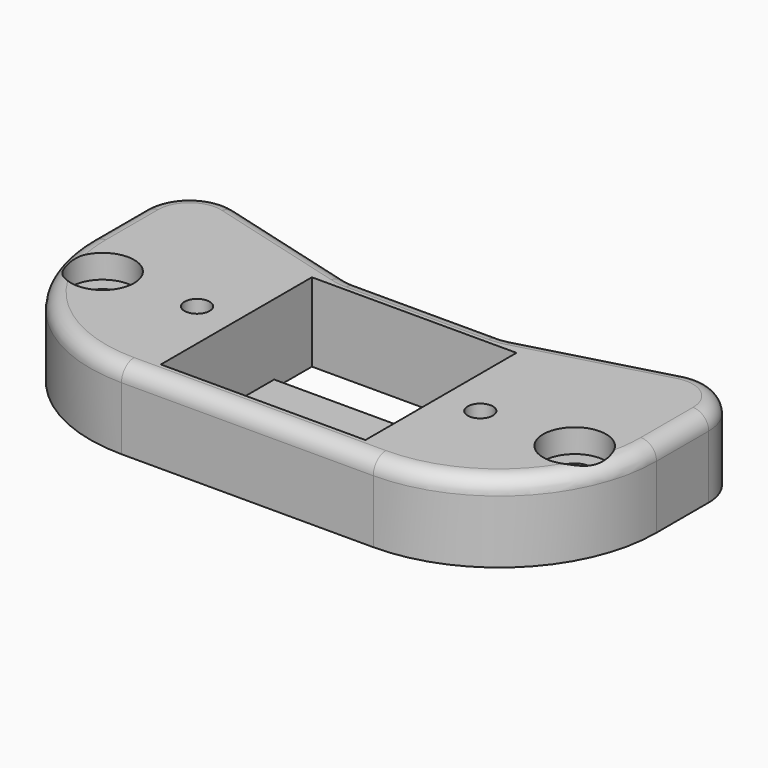
from build123d import *

# Parameters (mm, degrees)
F0_R           = 0.8
F0_W           = 13
F0_H           = 12
F1_DEPTH       = 5
F2_W           = 13
F2_H           = 6
F3_DEPTH       = 0.5
F5_D           = 2
F5_DEPTH       = 20
F5_CBORE_D     = 4
F5_CBORE_DEPTH = 1.5
F5_TIP         = 0.600860619
F6_R           = 10
F7_R           = 3
F8_T1_DEPTH    = 4.1430571099
F8_T3_DEPTH    = 9.217139142
F8_T5_DEPTH    = 16
F8_T7_DEPTH    = 9.0537269763
F8_T9_DEPTH    = 9.217139142
F8_T12_ANGLE   = 90
F8_T14_ANGLE   = 105.2904097565
F8_T16_ANGLE   = 90
F8_T18_ANGLE   = 15.2904100724
F8_T20_ANGLE   = 15.2904100724
F8_T22_ANGLE   = 105.2904094573


# Not quite as in the source:
# - a fillet or chamfer that OpenCascade refuses, or shapes differently, is made with other operations: its cross-section is extruded or revolved along the edge and cut away or added


with BuildPart() as f1:
    # F0 (on Top) → F1 (new body)
    with BuildSketch(Plane.XY):
        Polygon((-18, -7.25), (18, -7.25), (18, 7.25), (4.9295582736, 7.25), (-4.9295582736, 7.25), (-18, 7.25), align=None)
        with Locations((-9, 0)):
            Circle(F0_R, mode=Mode.SUBTRACT)
        Rectangle(F0_W, F0_H, mode=Mode.SUBTRACT)
        with Locations((9, 0)):
            Circle(F0_R, mode=Mode.SUBTRACT)
        with BuildLine():
            Line((4.9295582736, 7.25), (18, 7.25))
            ThreePointArc((18, 7.25), (17.6073787038, 9), (16.5047771245, 10.4145392323))
            Line((16.5047771245, 10.4145392323), (4.9295582736, 7.25))
        make_face()
        with BuildLine():
            ThreePointArc((-16.5047771245, 10.4145392323), (-17.6073787038, 9), (-18, 7.25))
            Line((-18, 7.25), (-4.9295582736, 7.25))
            Line((-4.9295582736, 7.25), (-16.5047771245, 10.4145392323))
        make_face()
    extrude(amount=F1_DEPTH)

    # F2 (on face) → F3 (join)
    with BuildSketch(Plane(origin=(0, 0, 0), x_dir=(1, 0, 0), z_dir=(0, 0, -1))):
        Rectangle(F2_W, F2_H)
    extrude(amount=-F3_DEPTH)

    # F5
    with Locations(Plane.XY.offset(5)):
        with Locations((-15, 0), (15, 0)):
            CounterBoreHole(F5_D / 2, F5_CBORE_D / 2, F5_CBORE_DEPTH, depth=F5_DEPTH)
            with Locations((0, 0, -(F5_DEPTH + F5_TIP / 2))):  # 118° drill point
                Cone(0, F5_D / 2, F5_TIP, mode=Mode.SUBTRACT)

    # F6
    f6_edges = [f1.edges().sort_by_distance(p)[0] for p in [
        (-18, -7.25, 2.5),
        (18, -7.25, 2.5),
    ]]
    fillet(f6_edges, radius=F6_R)

    # F7
    f7_edges = [f1.edges().sort_by_distance(p)[0] for p in [
        (-16.504777, 10.414539, 2.5),
        (16.504777, 10.414539, 2.5),
        (-4.929558, 7.25, 2.5),
        (4.929558, 7.25, 2.5),
    ]]
    fillet(f7_edges, radius=F7_R)

    # F8: fillet of radius 1 on 12 edges, made by hand

    # F8_s2 → F8_t1 (cut)
    with BuildSketch(Plane.XZ.offset(-6.8930571099)):
        with BuildLine():
            ThreePointArc((-18, 4), (-17.7071067812, 4.7071067812), (-17, 5))
            Line((-17, 5), (-18, 5))
            Line((-18, 5), (-18, 4))
        make_face()
        with BuildLine():
            ThreePointArc((18, 4), (17.7071067812, 4.7071067812), (17, 5))
            Line((17, 5), (18, 5))
            Line((18, 5), (18, 4))
        make_face()
    extrude(amount=F8_T1_DEPTH, mode=Mode.SUBTRACT)

    # F8_s4 → F8_t3 (cut)
    with BuildSketch(Plane(origin=(-6.8194085753, 1.8643523078, 0), x_dir=(0, 0, 1), z_dir=(-0.9646015709, 0.2637116027, 0))):
        with BuildLine():
            ThreePointArc((4, 5.6933796762), (4.7071067812, 5.4004864574), (5, 4.6933796762))
            Line((5, 4.6933796762), (5, 5.6933796762))
            Line((5, 5.6933796762), (4, 5.6933796762))
        make_face()
    extrude(amount=F8_T3_DEPTH, mode=Mode.SUBTRACT)

    # F8_s6 → F8_t5 (cut)
    with BuildSketch(Plane.YZ.offset(-8)):
        with BuildLine():
            ThreePointArc((-7.25, 4), (-6.9571067812, 4.7071067812), (-6.25, 5))
            Line((-6.25, 5), (-7.25, 5))
            Line((-7.25, 5), (-7.25, 4))
        make_face()
    extrude(amount=F8_T5_DEPTH, mode=Mode.SUBTRACT)

    # F8_s8 → F8_t7 (cut)
    with BuildSketch(Plane.YZ.offset(-4.5268634881)):
        with BuildLine():
            ThreePointArc((7.25, 4), (6.9571067812, 4.7071067812), (6.25, 5))
            Line((6.25, 5), (7.25, 5))
            Line((7.25, 5), (7.25, 4))
        make_face()
    extrude(amount=F8_T7_DEPTH, mode=Mode.SUBTRACT)

    # F8_s10 → F8_t9 (cut)
    with BuildSketch(Plane(origin=(15.7102754711, 4.2950188431, 0), x_dir=(0, 0, 1), z_dir=(-0.9646015709, -0.2637116027, 0))):
        with BuildLine():
            ThreePointArc((4, 5.6933796762), (4.7071067812, 5.4004864574), (5, 4.6933796762))
            Line((5, 4.6933796762), (5, 5.6933796762))
            Line((5, 5.6933796762), (4, 5.6933796762))
        make_face()
    extrude(amount=F8_T9_DEPTH, mode=Mode.SUBTRACT)

    # F8_s11 → F8_t12 (revolve, cut)
    with BuildSketch(Plane.YZ.offset(8)):
        with BuildLine():
            ThreePointArc((-7.25, 4), (-6.9571067812, 4.7071067812), (-6.25, 5))
            Line((-6.25, 5), (-7.25, 5))
            Line((-7.25, 5), (-7.25, 4))
        make_face()
    revolve(axis=Axis((8, 2.75, 5), (0, 0, 1)), revolution_arc=F8_T12_ANGLE, mode=Mode.SUBTRACT)

    # F8_s13 → F8_t14 (revolve, cut)
    with BuildSketch(Plane.XZ.offset(-6.8930571003)):
        with BuildLine():
            ThreePointArc((-18.0000000058, 4), (-17.707106787, 4.7071067812), (-17.0000000058, 5))
            Line((-17.0000000058, 5), (-18, 5))
            Line((-18, 5), (-18.0000000058, 4))
        make_face()
    revolve(axis=Axis((-14.9999999954, 6.8930571003, 5), (0, 0, -1)), revolution_arc=F8_T14_ANGLE, mode=Mode.SUBTRACT)

    # F8_s15 → F8_t16 (revolve, cut)
    with BuildSketch(Plane.YZ.offset(-8)):
        with BuildLine():
            ThreePointArc((-7.25, 4), (-6.9571067812, 4.7071067812), (-6.25, 5))
            Line((-6.25, 5), (-7.25, 5))
            Line((-7.25, 5), (-7.25, 4))
        make_face()
    revolve(axis=Axis((-8, 2.75, 5), (0, 0, -1)), revolution_arc=F8_T16_ANGLE, mode=Mode.SUBTRACT)

    # F8_s17 → F8_t18 (revolve, cut)
    with BuildSketch(Plane(origin=(-6.8194085753, 1.8643523078, 0), x_dir=(0, 0, 1), z_dir=(-0.9646015709, 0.2637116027, 0))):
        with BuildLine():
            ThreePointArc((4, 5.6933796762), (4.7071067812, 5.4004864574), (5, 4.6933796762))
            Line((5, 4.6933796762), (5, 5.6933796762))
            Line((5, 5.6933796762), (4, 5.6933796762))
        make_face()
    revolve(axis=Axis((-4.5268634881, 10.25, 5), (0, 0, 1)), revolution_arc=F8_T18_ANGLE, mode=Mode.SUBTRACT)

    # F8_s19 → F8_t20 (revolve, cut)
    with BuildSketch(Plane(origin=(6.8194085753, 1.8643523078, 0), x_dir=(0, 0, 1), z_dir=(0.9646015709, 0.2637116027, 0))):
        with BuildLine():
            ThreePointArc((4, -5.6933796762), (4.7071067812, -5.4004864574), (5, -4.6933796762))
            Line((5, -4.6933796762), (5, -5.6933796762))
            Line((5, -5.6933796762), (4, -5.6933796762))
        make_face()
    revolve(axis=Axis((4.5268634881, 10.25, 5), (0, 0, -1)), revolution_arc=F8_T20_ANGLE, mode=Mode.SUBTRACT)

    # F8_s21 → F8_t22 (revolve, cut)
    with BuildSketch(Plane.XZ.offset(-6.8930570951)):
        with BuildLine():
            ThreePointArc((18.0000000063, 4), (17.7071067875, 4.7071067812), (17.0000000063, 5))
            Line((17.0000000063, 5), (18, 5))
            Line((18, 5), (18.0000000063, 4))
        make_face()
    revolve(axis=Axis((14.999999986, 6.8930570951, 5), (0, 0, 1)), revolution_arc=F8_T22_ANGLE, mode=Mode.SUBTRACT)


solid = f1.part
